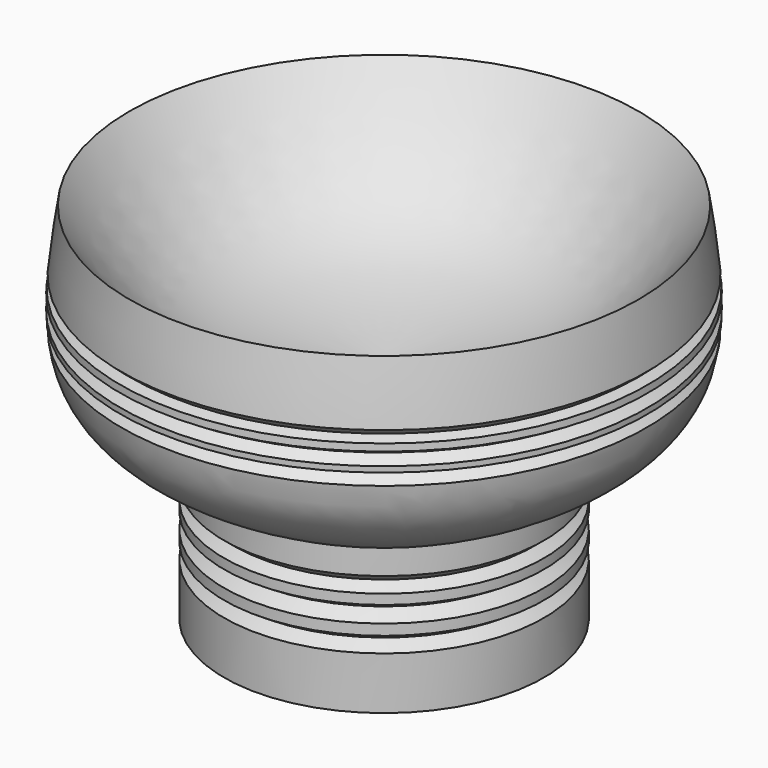
from build123d import *


with BuildPart() as f1:
    # F0 (on Front) → F1 (revolve)
    with BuildSketch(Plane.XZ):
        with BuildLine():
            Line((-11, 0), (-8.5, 0))
            Line((-8.5, 0), (-8.5, 11))
            Line((-8.5, 11), (0, 11))
            Line((0, 11), (0, 14.9984406307))
            add(Edge.make_bspline(
                [(-17.5161305815, 25.0157564878), (-15.5815870923, 22.2602219345), (-11.5737005689, 16.5514488505), (-3.9459538942, 15.5279254568), (0, 14.9984406307)],
                knots=[0, 0, 0, 0, 0.4826841973, 1, 1, 1, 1], degree=3))
            add(Edge.make_bspline(
                [(-18.072174276, 20.8134150085), (-17.9563486733, 22.1708113356), (-17.7362396274, 23.5932839117), (-17.5161305815, 25.0157564878)],
                knots=[0.7979590462, 0.7979590462, 0.7979590462, 0.7979590462, 1, 1, 1, 1], degree=3))
            Line((-18.072174276, 20.8134150085), (-17.474169231, 20.2877648349))
            Line((-17.474169231, 20.2877648349), (-18.1267939942, 20.0359687694))
            add(Edge.make_bspline(
                [(-18.1473092364, 19.552679753), (-18.1424496564, 19.7125412352), (-18.1355480675, 19.8736769971), (-18.1267939942, 20.0359687694)],
                knots=[0.7343469252, 0.7343469252, 0.7343469252, 0.7343469252, 0.7590029372, 0.7590029372, 0.7590029372, 0.7590029372], degree=3))
            Line((-18.1473092364, 19.552679753), (-17.5323307281, 19.1758368702))
            Line((-17.5323307281, 19.1758368702), (-18.1519210677, 18.6704946689))
            Line((-18.1519210677, 18.6704946689), (-18.1375525664, 18.2734475453))
            Line((-18.1375525664, 18.2734475453), (-17.5164529661, 17.9795547089))
            Line((-17.5164529661, 17.9795547089), (-18.06547265, 17.4323181276))
            add(Edge.make_bspline(
                [(-11, 10), (-13.635437822, 11.3804638315), (-17.0741854324, 13.1817078836), (-17.9594871723, 16.5763849323), (-18.06547265, 17.4323181276)],
                knots=[0, 0, 0, 0, 0.4755880726, 0.6205524314, 0.6205524314, 0.6205524314, 0.6205524314], degree=3))
            Line((-11, 10), (-11, 8.2959206775))
            Line((-11, 8.2959206775), (-10.267551057, 7.7029233798))
            Line((-10.267551057, 7.7029233798), (-11, 7.2285258211))
            Line((-11, 7.2285258211), (-11, 6.5465788357))
            Line((-11, 6.5465788357), (-10.1489517838, 6.0128816403))
            Line((-10.1489517838, 6.0128816403), (-11, 5.4198848084))
            Line((-11, 5.4198848084), (-11, 4.678638652))
            Line((-11, 4.678638652), (-10.1786013693, 4.144940991))
            Line((-10.1786013693, 4.144940991), (-11, 3.6112440284))
            Line((-11, 3.6112440284), (-11, 0))
        make_face()
    revolve(axis=Axis((0, 0, 7.4992203154), (0, 0, -1)))


solid = f1.part
